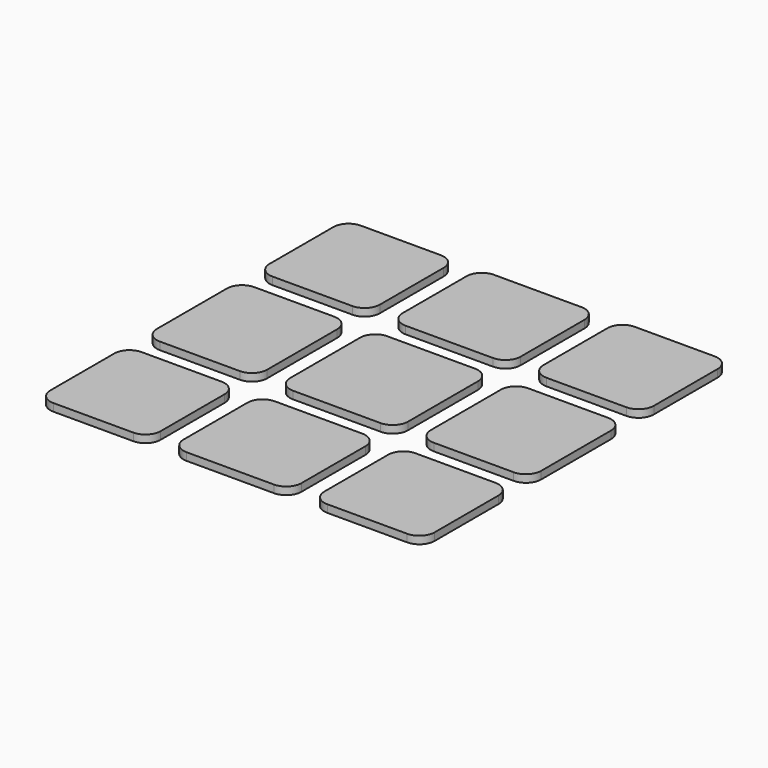
from build123d import *

# Parameters (mm, degrees)
F1_DEPTH = 1


with BuildPart() as f1:
    # F0 (on Top) → F1 (new body)
    with BuildSketch(Plane.XY):
        with BuildLine():
            Line((-12.75, -10.75), (-23.25, -10.75))
            ThreePointArc((-23.25, -10.75), (-24.6642135624, -11.3357864376), (-25.25, -12.75))
            Line((-25.25, -12.75), (-25.25, -23.25))
            ThreePointArc((-25.25, -23.25), (-24.6642135624, -24.6642135624), (-23.25, -25.25))
            Line((-23.25, -25.25), (-12.75, -25.25))
            ThreePointArc((-12.75, -25.25), (-11.3357864376, -24.6642135624), (-10.75, -23.25))
            Line((-10.75, -23.25), (-10.75, -12.75))
            ThreePointArc((-10.75, -12.75), (-11.3357864376, -11.3357864376), (-12.75, -10.75))
        make_face()
    extrude(amount=F1_DEPTH)


with BuildPart() as f1b:
    # F0 (on Top) → F1, piece 2 (new body)
    with BuildSketch(Plane.XY):
        with BuildLine():
            Line((5.75, -10.75), (-5.75, -10.75))
            ThreePointArc((-5.75, -10.75), (-7.1642135624, -11.3357864376), (-7.75, -12.75))
            Line((-7.75, -12.75), (-7.75, -23.25))
            ThreePointArc((-7.75, -23.25), (-7.1642135624, -24.6642135624), (-5.75, -25.25))
            Line((-5.75, -25.25), (5.75, -25.25))
            ThreePointArc((5.75, -25.25), (7.1642135624, -24.6642135624), (7.75, -23.25))
            Line((7.75, -23.25), (7.75, -12.75))
            ThreePointArc((7.75, -12.75), (7.1642135624, -11.3357864376), (5.75, -10.75))
        make_face()
    extrude(amount=F1_DEPTH)


with BuildPart() as f1c:
    # F0 (on Top) → F1, piece 3 (new body)
    with BuildSketch(Plane.XY):
        with BuildLine():
            ThreePointArc((7.75, 5.75), (7.1642135624, 7.1642135624), (5.75, 7.75))
            Line((5.75, 7.75), (-5.75, 7.75))
            ThreePointArc((-5.75, 7.75), (-7.1642135624, 7.1642135624), (-7.75, 5.75))
            Line((-7.75, 5.75), (-7.75, -5.75))
            ThreePointArc((-7.75, -5.75), (-7.1642135624, -7.1642135624), (-5.75, -7.75))
            Line((-5.75, -7.75), (5.75, -7.75))
            ThreePointArc((5.75, -7.75), (7.1642135624, -7.1642135624), (7.75, -5.75))
            Line((7.75, -5.75), (7.75, 5.75))
        make_face()
    extrude(amount=F1_DEPTH)


with BuildPart() as f1d:
    # F0 (on Top) → F1, piece 4 (new body)
    with BuildSketch(Plane.XY):
        with BuildLine():
            Line((10.75, 5.75), (10.75, -5.75))
            ThreePointArc((10.75, -5.75), (11.3357864376, -7.1642135624), (12.75, -7.75))
            Line((12.75, -7.75), (23.25, -7.75))
            ThreePointArc((23.25, -7.75), (24.6642135624, -7.1642135624), (25.25, -5.75))
            Line((25.25, -5.75), (25.25, 5.75))
            ThreePointArc((25.25, 5.75), (24.6642135624, 7.1642135624), (23.25, 7.75))
            Line((23.25, 7.75), (12.75, 7.75))
            ThreePointArc((12.75, 7.75), (11.3357864376, 7.1642135624), (10.75, 5.75))
        make_face()
    extrude(amount=F1_DEPTH)


with BuildPart() as f1e:
    # F0 (on Top) → F1, piece 5 (new body)
    with BuildSketch(Plane.XY):
        with BuildLine():
            ThreePointArc((10.75, -23.25), (11.3357864376, -24.6642135624), (12.75, -25.25))
            Line((12.75, -25.25), (23.25, -25.25))
            ThreePointArc((23.25, -25.25), (24.6642135624, -24.6642135624), (25.25, -23.25))
            Line((25.25, -23.25), (25.25, -12.75))
            ThreePointArc((25.25, -12.75), (24.6642135624, -11.3357864376), (23.25, -10.75))
            Line((23.25, -10.75), (12.75, -10.75))
            ThreePointArc((12.75, -10.75), (11.3357864376, -11.3357864376), (10.75, -12.75))
            Line((10.75, -12.75), (10.75, -23.25))
        make_face()
    extrude(amount=F1_DEPTH)


with BuildPart() as f1f:
    # F0 (on Top) → F1, piece 6 (new body)
    with BuildSketch(Plane.XY):
        with BuildLine():
            Line((-5.75, 10.75), (5.75, 10.75))
            ThreePointArc((5.75, 10.75), (7.1642135624, 11.3357864376), (7.75, 12.75))
            Line((7.75, 12.75), (7.75, 23.25))
            ThreePointArc((7.75, 23.25), (7.1642135624, 24.6642135624), (5.75, 25.25))
            Line((5.75, 25.25), (-5.75, 25.25))
            ThreePointArc((-5.75, 25.25), (-7.1642135624, 24.6642135624), (-7.75, 23.25))
            Line((-7.75, 23.25), (-7.75, 12.75))
            ThreePointArc((-7.75, 12.75), (-7.1642135624, 11.3357864376), (-5.75, 10.75))
        make_face()
    extrude(amount=F1_DEPTH)


with BuildPart() as f1g:
    # F0 (on Top) → F1, piece 7 (new body)
    with BuildSketch(Plane.XY):
        with BuildLine():
            ThreePointArc((23.25, 10.75), (24.6642135624, 11.3357864376), (25.25, 12.75))
            Line((25.25, 12.75), (25.25, 23.25))
            ThreePointArc((25.25, 23.25), (24.6642135624, 24.6642135624), (23.25, 25.25))
            Line((23.25, 25.25), (12.75, 25.25))
            ThreePointArc((12.75, 25.25), (11.3357864376, 24.6642135624), (10.75, 23.25))
            Line((10.75, 23.25), (10.75, 12.75))
            ThreePointArc((10.75, 12.75), (11.3357864376, 11.3357864376), (12.75, 10.75))
            Line((12.75, 10.75), (23.25, 10.75))
        make_face()
    extrude(amount=F1_DEPTH)


with BuildPart() as f1h:
    # F0 (on Top) → F1, piece 8 (new body)
    with BuildSketch(Plane.XY):
        with BuildLine():
            Line((-10.75, -5.75), (-10.75, 5.75))
            ThreePointArc((-10.75, 5.75), (-11.3357864376, 7.1642135624), (-12.75, 7.75))
            Line((-12.75, 7.75), (-23.25, 7.75))
            ThreePointArc((-23.25, 7.75), (-24.6642135624, 7.1642135624), (-25.25, 5.75))
            Line((-25.25, 5.75), (-25.25, -5.75))
            ThreePointArc((-25.25, -5.75), (-24.6642135624, -7.1642135624), (-23.25, -7.75))
            Line((-23.25, -7.75), (-12.75, -7.75))
            ThreePointArc((-12.75, -7.75), (-11.3357864376, -7.1642135624), (-10.75, -5.75))
        make_face()
    extrude(amount=F1_DEPTH)


with BuildPart() as f1i:
    # F0 (on Top) → F1, piece 9 (new body)
    with BuildSketch(Plane.XY):
        with BuildLine():
            ThreePointArc((-10.75, 23.25), (-11.3357864376, 24.6642135624), (-12.75, 25.25))
            Line((-12.75, 25.25), (-23.25, 25.25))
            ThreePointArc((-23.25, 25.25), (-24.6642135624, 24.6642135624), (-25.25, 23.25))
            Line((-25.25, 23.25), (-25.25, 12.75))
            ThreePointArc((-25.25, 12.75), (-24.6642135624, 11.3357864376), (-23.25, 10.75))
            Line((-23.25, 10.75), (-12.75, 10.75))
            ThreePointArc((-12.75, 10.75), (-11.3357864376, 11.3357864376), (-10.75, 12.75))
            Line((-10.75, 12.75), (-10.75, 23.25))
        make_face()
    extrude(amount=F1_DEPTH)


solid = Compound([f1.part, f1b.part, f1c.part, f1d.part, f1e.part, f1f.part, f1g.part, f1h.part, f1i.part])
